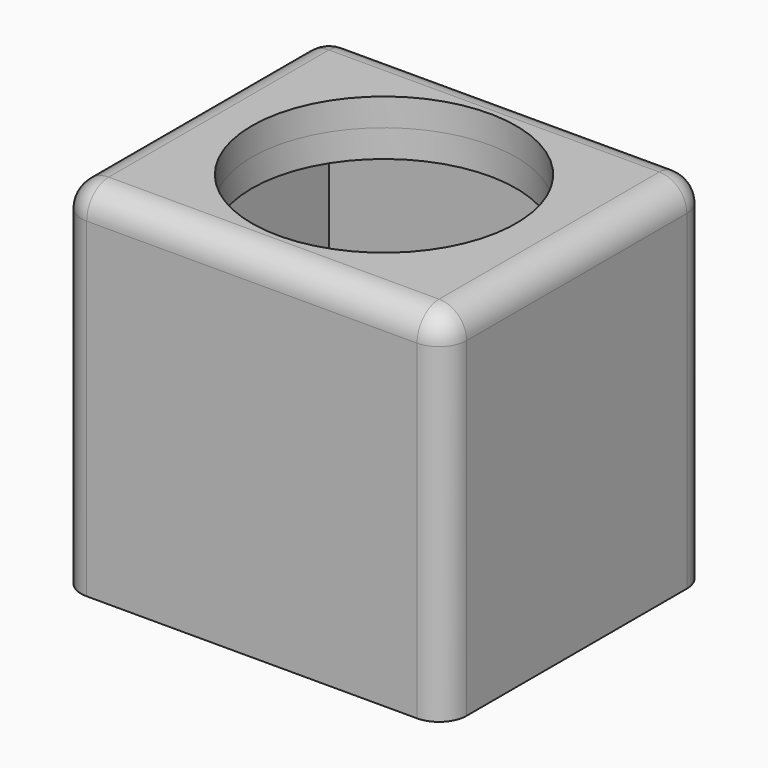
from build123d import *

# Parameters (mm, degrees)
F1_DEPTH = 60
F2_W     = 70
F2_H     = 5
F3_DEPTH = 60
F5_D     = 48
F6_R     = 4.99999
F6_2_R   = 4.99999
F7_T     = 5
F8_D     = 48


# Not quite as in the source:
# - a fillet or chamfer is up to 0.001 mm smaller than in the source, because OpenCascade refuses the exact size
# - a shell that OpenCascade refuses in one call is made with other operations: the cavity is built on its own and cut out
# - a feature names something its author has since deleted; it is built from what else it names


with BuildPart() as f1:
    # F0 (on Top) → F1 (new body)
    with BuildSketch(Plane.XY):
        Polygon((10, 0), (0, 0), (0, -10), (0, -50), (0, -60), (10, -60), (60, -60), (70, -60), (70, -50), (70, -10), (70, 0), (60, 0), align=None)
    extrude(amount=F1_DEPTH)

    # F6#2 (radius 5 in the source; OpenCascade refuses exactly that, so slightly less here)
    f6_2_edges = [f1.edges().sort_by_distance(p)[0] for p in [
        (0, -60, 30),
        (70, -60, 30),
        (70, 0, 30),
        (0, 0, 30),
    ]]
    fillet(f6_2_edges, radius=F6_2_R)

    # F7: shell of thickness 5, made by hand


with BuildPart() as f3:
    # F2 (on Front) → F3 (new body)
    with BuildSketch(Plane.XZ):
        with Locations((35, 62.5)):
            Rectangle(F2_W, F2_H)
    extrude(amount=F3_DEPTH)

    # F5 (through all)
    with Locations(Plane.XY.offset(65)):
        with Locations((35, -30)):
            Hole(F5_D / 2)

    # F6 (radius 5 in the source; OpenCascade refuses exactly that, so slightly less here)
    f6_edges = [f3.edges().sort_by_distance(p)[0] for p in [
        (0, -30, 65),
        (35, 0, 65),
        (70, -30, 65),
        (35, -60, 65),
        (0, 0, 62.5),
        (0, -60, 62.5),
        (70, 0, 62.5),
        (70, -60, 62.5),
    ]]
    fillet(f6_edges, radius=F6_R)


with BuildPart() as f7_core1:
    # F7_t2: copy of F1
    add(f1.part)

    # the walls: a layer under each face that stays
    f7_faces = [f7_core1.faces().sort_by_distance(p)[0] for p in [
        (35, 0, 30),
        (35, -30, 60),
        (0, -30, 30),
        (35, -60, 30),
        (70, -30, 30),
    ]]
    thicken(f7_faces, amount=-F7_T, mode=Mode.SUBTRACT)


with BuildPart() as f1_1:
    add(f1.part)

    # what is left inside the walls is the cavity
    f7_cavity = [f7_core1.part.solids().sort_by_distance(p)[0] for p in [
        (35, -5.05, 36.666667),
    ]]
    add(f7_cavity, mode=Mode.SUBTRACT)

    # F8 (through all)
    with Locations(Plane.XY.offset(65)):
        with Locations((35, -30)):
            Hole(F8_D / 2)


solid = Compound([f3.part, f1_1.part])
